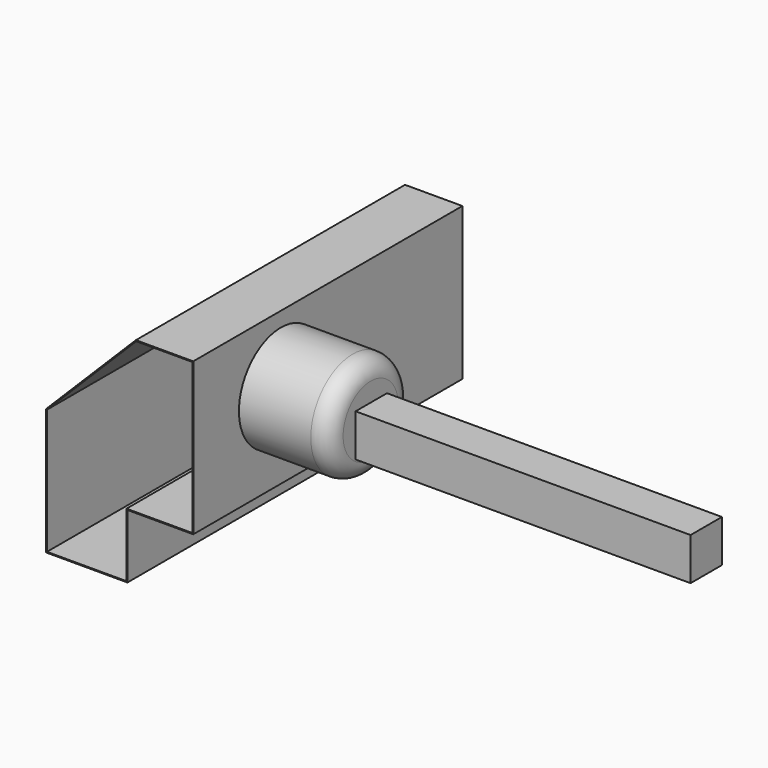
from build123d import *

# Parameters (mm, degrees)
F1_DEPTH  = 95.1442476362
F4_SIZE   = 25.4
F5_T      = -0.254
F7_R      = 14.8113832011
F8_DEPTH  = 25.4
F9_W      = 11.0863484442
F9_H      = 11.992841959
F10_DEPTH = 94.742
F11_R     = 5.08


# Not quite as in the source:
# - the program builds the solid bodies; features that only make, move or delete a surface that nothing else refers to are left out


with BuildPart() as f1:
    # F0 (on Front) → F1 (new body)
    with BuildSketch(Plane.XZ):
        Polygon((-9.3385055661, 8.2524567842), (13.6685147882, 8.2524567842), (13.6685147882, 26.3094156981), (32.2877131402, 26.3094156981), (32.2877131402, 69.3843364716), (-9.3385055661, 69.3843364716), align=None)
    extrude(amount=F1_DEPTH)

    # F4
    f4_edges = [f1.edges().sort_by_distance(p)[0] for p in [
        (-9.338506, -47.572124, 69.384336),
    ]]
    chamfer(f4_edges, length=F4_SIZE)

    # F5
    f5_openings = [f1.faces().sort_by_distance(p)[0] for p in [
        (11.53567, -95.144248, 38.877913),
    ]]
    offset(amount=F5_T, openings=f5_openings, kind=Kind.INTERSECTION)

    # F7 (on face) → F8 (join)
    with BuildSketch(Plane.YZ.offset(32.2877131402)):
        with Locations((-64.1838386655, 50.4019707441)):
            Circle(F7_R)
    extrude(amount=F8_DEPTH)

    # F9 (on face) → F10 (join)
    with BuildSketch(Plane.YZ.offset(57.6877131402)):
        with Locations((-63.960975036, 48.7824268639)):
            Rectangle(F9_W, F9_H)
    extrude(amount=F10_DEPTH)

    # F11
    f11_edges = [f1.edges().sort_by_distance(p)[0] for p in [
        (57.687713, -78.995222, 50.401971),
    ]]
    fillet(f11_edges, radius=F11_R)


solid = f1.part
